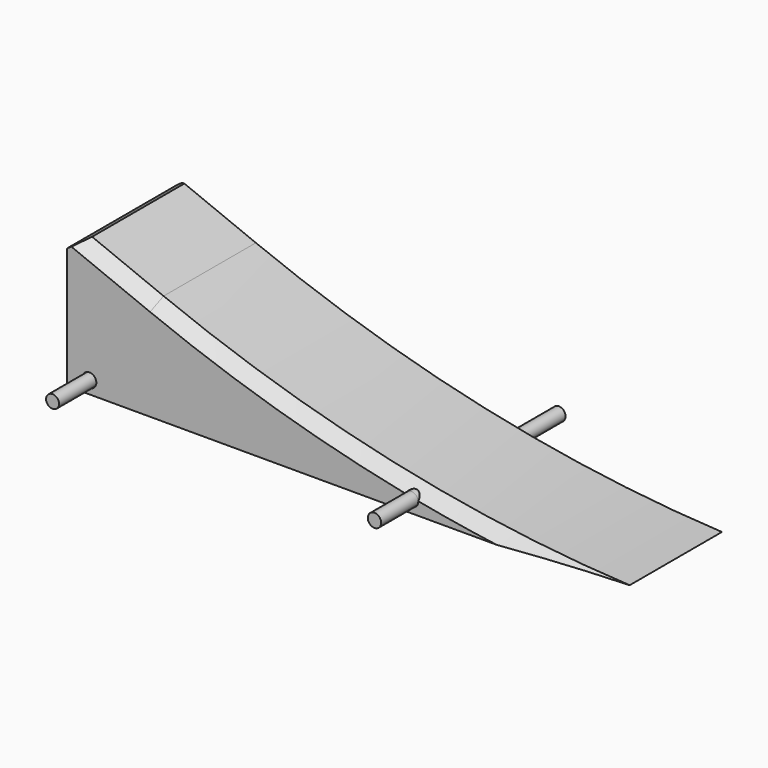
from build123d import *

# Parameters (mm, degrees)
F1_DEPTH    = 76.2
F2_R        = 3.81
F3_DEPTH    = 76.2
F4_T1_DEPTH = 68.223556095
F4_T3_DEPTH = 124.0305188657
F4_T6_ANGLE = 20.3486989559
F4_T8_ANGLE = 20.3486989559
F5_R        = 3.5695769538
F6_DEPTH    = 101.6
F5_R_2      = 3.6795438925
F6_FACE_R   = 3.5695769538
F7_DEPTH    = 25.4
F8_DEPTH    = 101.6


# Not quite as in the source:
# - a fillet or chamfer that OpenCascade refuses, or shapes differently, is made with other operations: its cross-section is extruded or revolved along the edge and cut away or added


with BuildPart() as f1:
    # F0 (on Front) → F1 (new body)
    with BuildSketch(Plane.XZ):
        with BuildLine():
            Line((-317.2810375895, 0), (-12.4810375895, 0))
            ThreePointArc((-12.4810375895, 0), (-143.2080739486, 17.6048536016), (-269.1808342934, 56.7245744169))
            Line((-269.1808342934, 56.7245744169), (-317.2810375895, 76.2))
            Line((-317.2810375895, 76.2), (-317.2810375895, 0))
        make_face()
    extrude(amount=F1_DEPTH)

    # F2 (on face) → F3 (cut)
    with BuildSketch(Plane.XZ.offset(76.2)):
        with Locations((-304.942605689, 6.888254699)):
            Circle(F2_R)
        with Locations((-127.6531666517, 6.8997577764)):
            Circle(F2_R)
    extrude(amount=-F3_DEPTH, mode=Mode.SUBTRACT)

    # F4: chamfer of 6.35 on 5 edges, made by hand

    # F4_s2 → F4_t1 (cut)
    with BuildSketch(Plane(origin=(-250.9997630926, 0, 101.6279947383), x_dir=(0, 1, 0), z_dir=(-0.9269046144, 0, 0.3752969968))):
        Polygon((-6.35, 48.4444889184), (0, 54.7944889184), (0, 48.4444889184), align=None)
        Polygon((-69.85, 48.4444889184), (-76.2, 54.7944889184), (-76.2, 48.4444889184), align=None)
    extrude(amount=F4_T1_DEPTH, mode=Mode.SUBTRACT)

    # F4_s4 → F4_t3 (cut)
    with BuildSketch(Plane.XZ.offset(-23.9152594329)):
        Polygon((-308.5479016601, 72.6640162152), (-317.2810375895, 66.7781719137), (-317.2810375895, 76.2), align=None)
    extrude(amount=F4_T3_DEPTH, mode=Mode.SUBTRACT)

    # F4_s5 → F4_t6 (revolve, cut)
    with BuildSketch(Plane(origin=(3.8520530857, 0, -0.1139205939), x_dir=(0, 1, 0), z_dir=(0.9995629761, 0, -0.0295610692))):
        Polygon((-69.85, -0.5378053162), (-76.2, -6.8878053162), (-76.2, -0.5378053162), align=None)
    revolve(axis=Axis((27.1796188092, -76.2, 788.6725353144), (0, 1, 0)), revolution_arc=F4_T6_ANGLE, mode=Mode.SUBTRACT)

    # F4_s7 → F4_t8 (revolve, cut)
    with BuildSketch(Plane(origin=(3.8520530857, 0, -0.1139205939), x_dir=(0, 1, 0), z_dir=(0.9995629761, 0, -0.0295610692))):
        Polygon((-6.35, -0.5378053162), (0, -6.8878053162), (0, -0.5378053162), align=None)
    revolve(axis=Axis((27.1796188092, 0, 788.6725353144), (0, 1, 0)), revolution_arc=F4_T8_ANGLE, mode=Mode.SUBTRACT)


with BuildPart() as f6:
    # F5 (on face) → F6 (new body)
    with BuildSketch(Plane.XZ.offset(76.2)):
        with Locations((-304.942605689, 6.888254699)):
            Circle(F5_R)
    extrude(amount=-F6_DEPTH)

    # F5 (on face) + F6_face (on face) → F7 (join)
    with BuildSketch(Plane.XZ.offset(76.2)):
        with Locations((-304.942605689, 6.888254699)):
            Circle(F5_R)
        with Locations((-127.6531666517, 6.8997577764)):
            Circle(F5_R_2)
    with BuildSketch(Plane(origin=(-304.942605689, -76.2, 6.888254699), x_dir=(1, 0, 0), z_dir=(0, -1, 0))):
        Circle(F6_FACE_R)
    extrude(amount=F7_DEPTH)


with BuildPart() as f8:
    # F5 (on face) → F8 (new body)
    with BuildSketch(Plane.XZ.offset(76.2)):
        with Locations((-304.942605689, 6.888254699)):
            Circle(F5_R)
    extrude(amount=-F8_DEPTH)


with BuildPart() as f8b:
    # F5 (on face) → F8, piece 2 (new body)
    with BuildSketch(Plane.XZ.offset(76.2)):
        with Locations((-127.6531666517, 6.8997577764)):
            Circle(F5_R_2)
    extrude(amount=-F8_DEPTH)


solid = Compound([f1.part, f6.part, f8.part, f8b.part])
